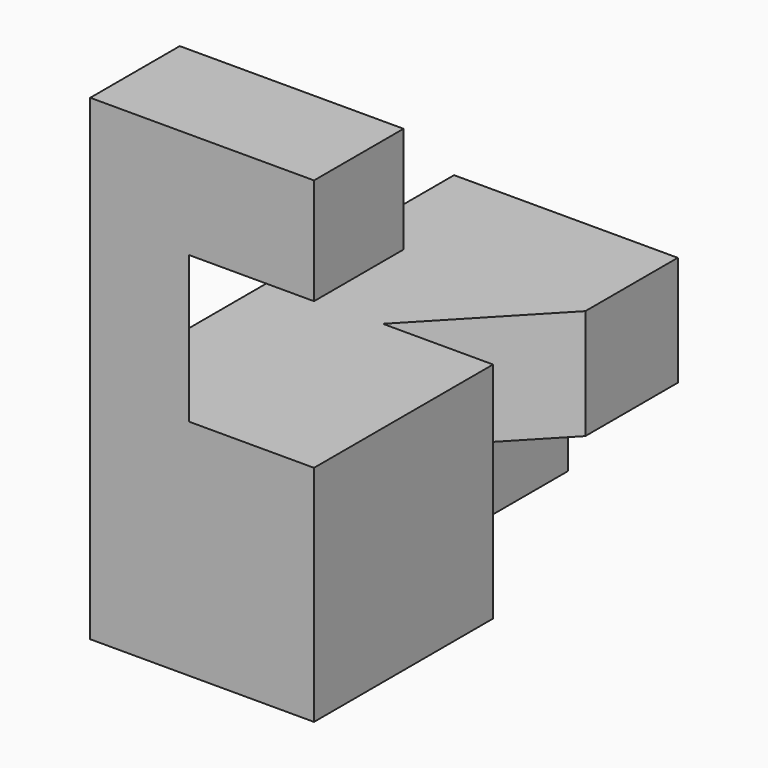
from build123d import *

# Parameters (mm, degrees)
F0_W      = 15.5
F0_H      = 15.5
F1_DEPTH  = 7.747
F3_DEPTH  = 10.16
F4_W      = 15.5
F4_H      = 7.75
F5_DEPTH  = 7.366
F6_W      = 7.874
F6_H      = 15.494
F7_DEPTH  = 16.002
F8_W      = 8.001
F8_H      = 7.62
F9_DEPTH  = 7.62
F11_DEPTH = 7.62


with BuildPart() as f1:
    # F0 (on Top) → F1 (new body, symmetric)
    with BuildSketch(Plane.XY):
        Rectangle(F0_W, F0_H)
    extrude(amount=F1_DEPTH, both=True)

    # F2 (on face) → F3 (join)
    with BuildSketch(Plane.XY.offset(7.747)):
        Polygon((-7.75, -0.384), (-7.75, -7.75), (-0.892, -7.75), align=None)
    extrude(amount=F3_DEPTH)

    # F4 (on face) → F5 (join)
    with BuildSketch(Plane.XY.offset(17.907)):
        with Locations((0, -3.875)):
            Rectangle(F4_W, F4_H)
    extrude(amount=F5_DEPTH)

    # F6 (on face) → F7 (join)
    with BuildSketch(Plane(origin=(0, 7.75, 0), x_dir=(-1, 0, 0), z_dir=(0, 1, 0))):
        with Locations((3.813, 0)):
            Rectangle(F6_W, F6_H)
    extrude(amount=F7_DEPTH)

    # F8 (on face) → F9 (join)
    with BuildSketch(Plane.YZ.offset(0.124)):
        with Locations((19.7515, 3.937)):
            Rectangle(F8_W, F8_H)
    extrude(amount=F9_DEPTH)

    # F10 (on face) → F11 (join)
    with BuildSketch(Plane.XY.offset(7.747)):
        Polygon((0.124, 7.75), (7.744, 15.751), (0.124, 15.751), align=None)
    extrude(amount=-F11_DEPTH)


solid = f1.part
